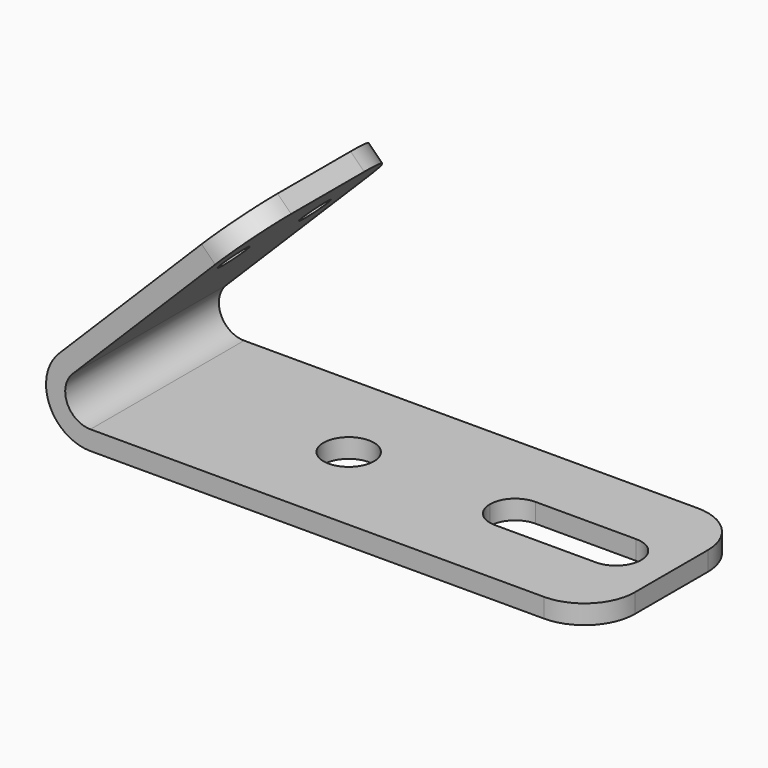
from build123d import *

# Parameters (mm, degrees)
F1_DEPTH = 190.5
F2_R     = 50
F3_R     = 25
F4_DEPTH = 25
F5_DEPTH = 25
F6_R     = 15
F7_DEPTH = 25


# Not quite as in the source:
# - ends of sketch curves that miss each other by under 0.0002 mm in the source are joined


with BuildPart() as f1:
    # F0 (on Front) → F1 (new body)
    with BuildSketch(Plane.XZ):
        with BuildLine():
            Line((145.6639969244, 207.8893936688), (-31.1126983722, 31.1126983722))
            ThreePointArc((-31.1126983722, 31.1126983722), (-40.6506994305, -16.8380710241), (0, -44))
            Line((0, -44), (500, -44))
            Line((500, -44), (500, -25))
            Line((500, -25), (0, -24.9999985185))
            ThreePointArc((0, -24.9999985185), (-23.096986944, -9.5670852422), (-17.6776684821, 17.6776684821))
            Line((-17.6776684821, 17.6776684821), (159.0990268146, 194.4543637787))
            Line((159.0990268146, 194.4543637787), (145.6639969244, 207.8893936688))
        make_face()
    extrude(amount=F1_DEPTH)

    # F2
    f2_edges = [f1.edges().sort_by_distance(p)[0] for p in [
        (500, 0, -34.5),
        (500, -190.5, -34.5),
        (152.381512, -190.5, 201.171879),
        (152.381512, 0, 201.171879),
    ]]
    fillet(f2_edges, radius=F2_R)

    # F3 (on face) → F4 (cut)
    with BuildSketch(Plane.XY.offset(-24.9999985185)):
        with Locations((180, -95.25)):
            Circle(F3_R)
    extrude(amount=-F4_DEPTH, mode=Mode.SUBTRACT)

    # F3 (on face) → F5 (cut)
    with BuildSketch(Plane.XY.offset(-24.9999985185)):
        with BuildLine():
            Line((445.0901150703, -70.25), (345.0901150703, -70.25))
            ThreePointArc((345.0901150703, -70.25), (327.4124455407, -77.5723304703), (320.0901150703, -95.25))
            ThreePointArc((320.0901150703, -95.25), (327.4124455407, -112.9276695297), (345.0901150703, -120.25))
            Line((345.0901150703, -120.25), (445.0901150703, -120.25))
            ThreePointArc((445.0901150703, -120.25), (462.7677846, -112.9276695297), (470.0901150703, -95.25))
            ThreePointArc((470.0901150703, -95.25), (462.7677846, -77.5723304703), (445.0901150703, -70.25))
        make_face()
    extrude(amount=-F5_DEPTH, mode=Mode.SUBTRACT)

    # F6 (on face) → F7 (cut)
    with BuildSketch(Plane(origin=(-31.1126983722, 0, 31.1126983722), x_dir=(0, -1, 0), z_dir=(-0.7071067812, 0, 0.7071067812))):
        with Locations((45, 175)):
            Circle(F6_R)
        with Locations((145.5, 175)):
            Circle(F6_R)
    extrude(amount=-F7_DEPTH, mode=Mode.SUBTRACT)


solid = f1.part
